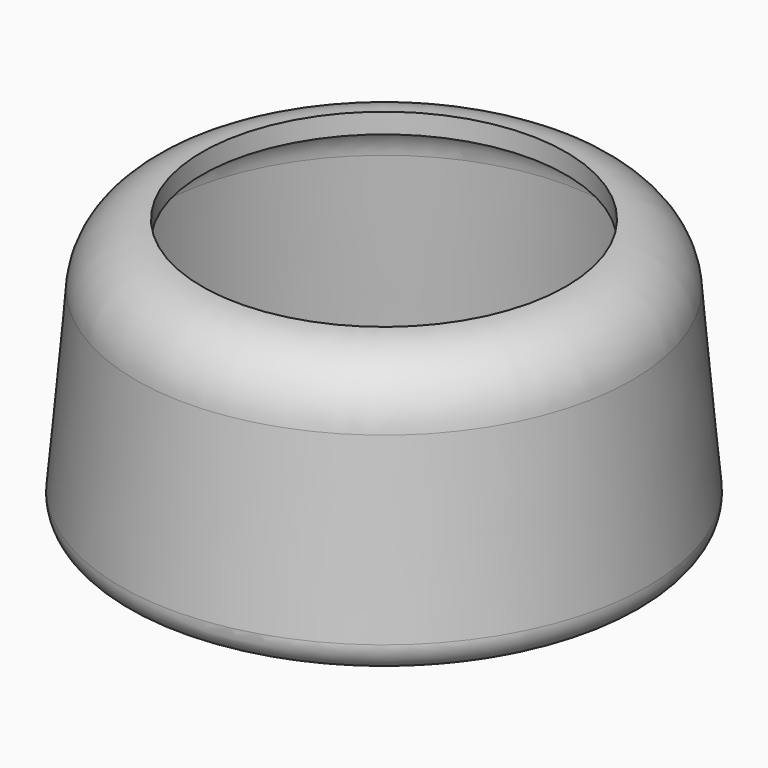
from build123d import *

# Parameters (mm, degrees)
F0_R     = 50.8
F1_DEPTH = 50.8
F1_TAPER = 5
F2_R     = 12.7
F3_T     = -3.81
F4_R     = 2.54
F6_D     = 7.62
F7_R     = 5.08


# Not quite as in the source:
# - a shell that OpenCascade refuses in one call is made with other operations: the cavity is built on its own and cut out


with BuildPart() as f1:
    # F0 (on Top) → F1 (new body)
    with BuildSketch(Plane.XY):
        Circle(F0_R)
    extrude(amount=F1_DEPTH, taper=F1_TAPER)

    # F2
    f2_edges = [f1.edges().sort_by_distance(p)[0] for p in [
        (-46.355576, 0, 50.8),
    ]]
    fillet(f2_edges, radius=F2_R)

    # F3: a shell. OpenCascade refuses it in one call, so the cavity is built on its own and cut out:
    # the body offset inwards by the wall thickness, plus a prism from it out through each open face.
    f3_core = offset(f1.part, amount=F3_T, mode=Mode.PRIVATE)
    f3_exits = [f3_core.faces().sort_by_distance(p)[0] for p in [
        (0, 0, 46.99),
    ]]
    add(f3_core, mode=Mode.SUBTRACT)
    extrude(f3_exits, amount=-F3_T, mode=Mode.SUBTRACT)

    # F4
    f4_edges = [f1.edges().sort_by_distance(p)[0] for p in [
        (-46.642115, 0, 3.81),
    ]]
    fillet(f4_edges, radius=F4_R)

    # F6 (through all)
    with Locations(Plane(origin=(0, 0, 0), x_dir=(1, 0, 0), z_dir=(0, 0, -1))):
        with Locations((3.3266340716, -15.1329960019), (-11.4422419373, -10.4474476161), (-14.7688760089, 4.6855483859), (-3.3266340716, 15.1329960019), (11.4422419373, 10.4474476161), (14.7688760089, -4.6855483859), (0, 0)):
            Hole(F6_D / 2)

    # F7
    f7_edges = [f1.edges().sort_by_distance(p)[0] for p in [
        (-50.8, 0, 0),
    ]]
    fillet(f7_edges, radius=F7_R)


solid = f1.part
